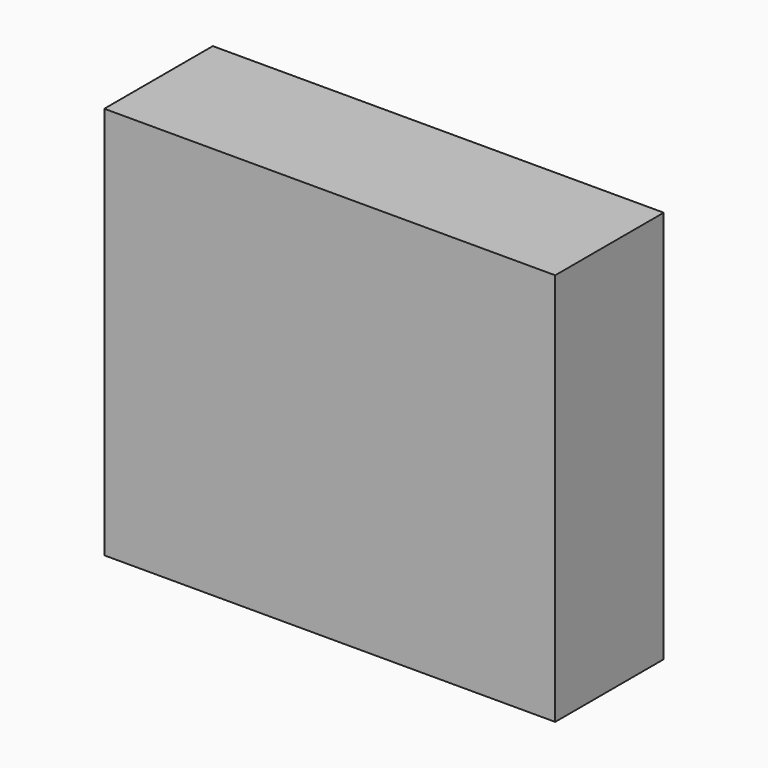
from build123d import *

# Parameters (mm, degrees)
F0_W     = 84.4428054988
F0_H     = 73.6313704401
F1_DEPTH = 25.4


# Not quite as in the source:
# - the program builds the solid bodies; features that only make, move or delete a surface that nothing else refers to are left out


with BuildPart() as f1:
    # F0 (on Front) → F1 (new body)
    with BuildSketch(Plane.XZ):
        with Locations((-16.9563870877, 8.6702173576)):
            Rectangle(F0_W, F0_H)
    extrude(amount=F1_DEPTH)


solid = f1.part
